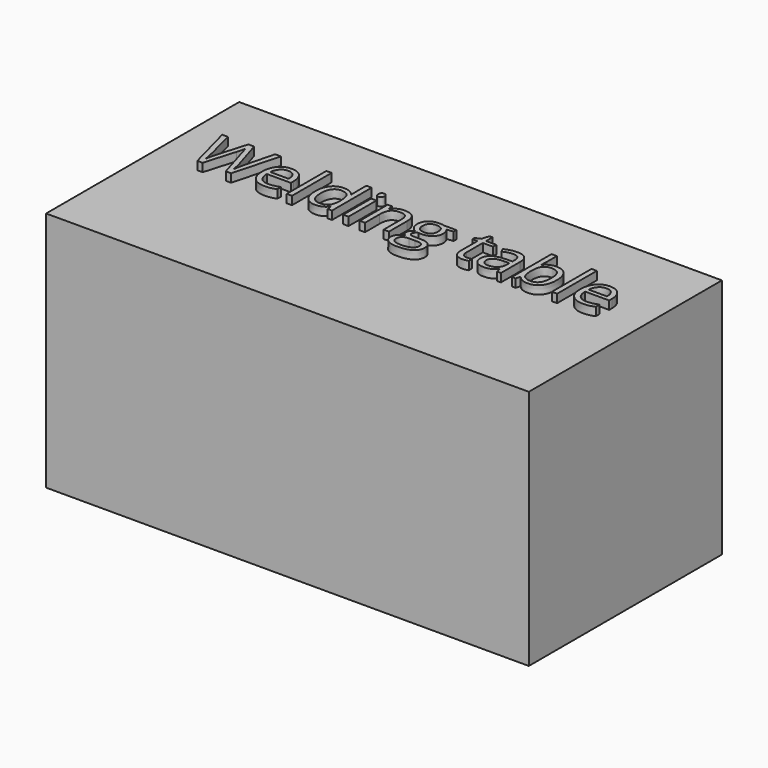
from build123d import *

# Parameters (mm, degrees)
F0_W         = 1473.2
F0_H         = 736.6
F1_DEPTH     = 736.6
F2_TEXT_SIZE = 199.2010391393
F3_DEPTH     = 25.4


# Not quite as in the source:
# - Text() gives the source's letters only with a copy of the font that has no kerning and outlines rounded to 1/6400 em; it was checked with that copy


with BuildPart() as f1:
    # F0 (on Top) → F1 (new body)
    with BuildSketch(Plane.XY):
        Rectangle(F0_W, F0_H)
    extrude(amount=F1_DEPTH)

    # F2 (on face) → F3 (join)
    with BuildSketch(Plane.XY.offset(736.6)):
        with Locations((-635, 30.9404211195)):
            Text('Welding table', F2_TEXT_SIZE, font='Open Sans', text_align=(TextAlign.LEFT, TextAlign.BOTTOM))
    extrude(amount=F3_DEPTH)


solid = f1.part
